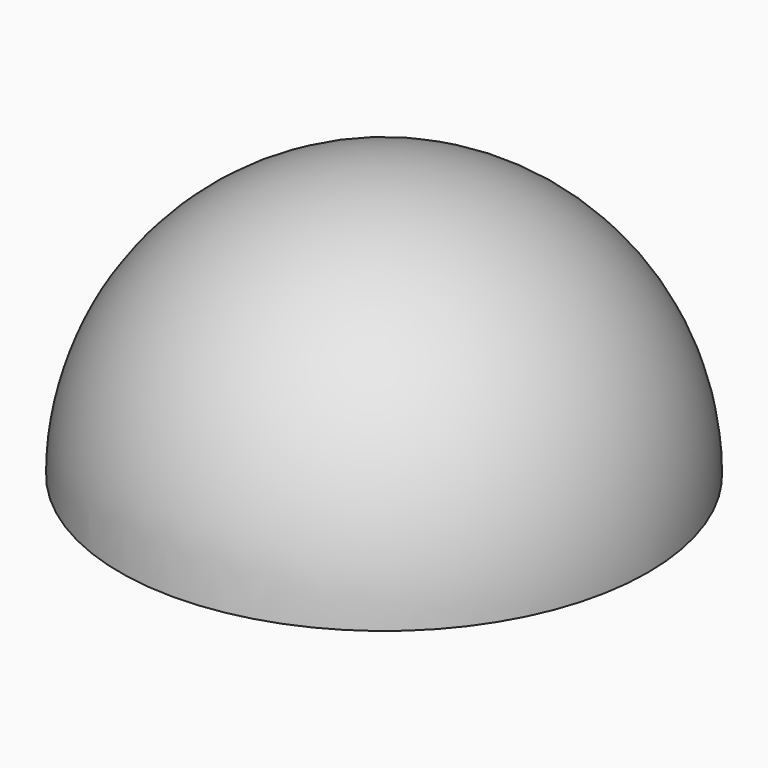
from build123d import *

# Parameters (mm, degrees)
F2_ANGLE     = 180
F0_R         = 2.54
F3_DEPTH     = 2.54
F4_R         = 1.5875
F5_DEPTH     = 25.4
F6_TEXT_SIZE = 4.0643677523
F7_DEPTH     = 0.508
F8_TEXT_SIZE = 8.6958589339
F9_DEPTH     = 0.508


# Not quite as in the source:
# - Text() gives the source's letters only with a copy of the font that has no kerning and outlines rounded to 1/6400 em; it was checked with that copy


with BuildPart() as f2:
    # F1 (on Top) → F2 (revolve)
    with BuildSketch(Plane.XY):
        with BuildLine():
            ThreePointArc((12.7, 0), (0, 12.7), (-12.7, 0))
            Line((-12.7, 0), (12.7, 0))
        make_face()
    revolve(axis=Axis((0, 0, 0), (1, 0, 0)), revolution_arc=F2_ANGLE)

    # F0 (on Top) → F3 (join)
    with BuildSketch(Plane.XY):
        with Locations((-6.0204306359, 11.1823260084)):
            Circle(F0_R)
    extrude(amount=F3_DEPTH)

    # F4 (on face) → F5 (cut)
    with BuildSketch(Plane.XY.offset(2.54)):
        with Locations((-6.0204306359, 11.1823260084)):
            Circle(F4_R)
    extrude(amount=-F5_DEPTH, mode=Mode.SUBTRACT)

    # F6 (on face) → F7 (cut)
    with BuildSketch(Plane(origin=(0, 0, 0), x_dir=(1, 0, 0), z_dir=(0, 0, -1))):
        with Locations((-6.6721637415, 4.2922910866)):
            Text('Lobos', F6_TEXT_SIZE, font='Open Sans', font_style=FontStyle.BOLD, text_align=(TextAlign.LEFT, TextAlign.BOTTOM))
        with Locations((-10.896565974, -1.2352490565)):
            Text('Basketball', F6_TEXT_SIZE, font='Open Sans', font_style=FontStyle.BOLD, text_align=(TextAlign.LEFT, TextAlign.BOTTOM))
    extrude(amount=-F7_DEPTH, mode=Mode.SUBTRACT)

    # F8 (on face) → F9 (cut)
    with BuildSketch(Plane(origin=(0, 0, 0), x_dir=(1, 0, 0), z_dir=(0, 0, -1))):
        with Locations((-7.4797522646, -10.4223696366)):
            Text('#31', F8_TEXT_SIZE, font='Open Sans', font_style=FontStyle.BOLD, text_align=(TextAlign.LEFT, TextAlign.BOTTOM))
    extrude(amount=-F9_DEPTH, mode=Mode.SUBTRACT)


solid = f2.part
